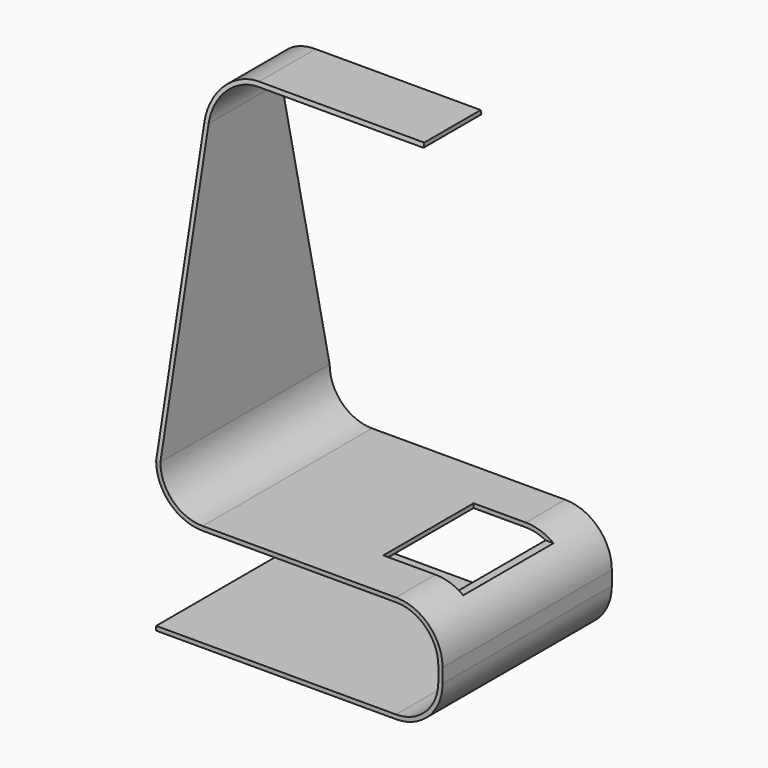
from build123d import *

# Parameters (mm, degrees)
F1_DEPTH = 75
F3_DEPTH = 200
F4_W     = 37
F4_H     = 40
F4_W_2   = 33
F5_DEPTH = 6.5


# Not quite as in the source:
# - a feature names something its author has since deleted; it is built from what else it names


with BuildPart() as f1:
    # F0 (on Front) → F1 (new body, symmetric)
    with BuildSketch(Plane.XZ):
        with BuildLine():
            Line((-67, 35), (70, 35))
            ThreePointArc((70, 35), (91.2132034356, 26.2132034356), (100, 5))
            Line((100, 5), (100, -5))
            ThreePointArc((100, -5), (91.2132034356, -26.2132034356), (70, -35))
            Line((70, -35), (-100, -35))
            Line((-100, -35), (-100, -38))
            Line((-100, -38), (70, -38))
            ThreePointArc((70, -38), (93.3345237792, -28.3345237792), (103, -5))
            Line((103, -5), (103, 5))
            ThreePointArc((103, 5), (93.3345237792, 28.3345237792), (70, 38))
            Line((70, 38), (-67, 38))
            ThreePointArc((-67, 38), (-88.2132034356, 46.7867965644), (-97, 68))
            Line((-97, 68), (-97, 262))
            ThreePointArc((-97, 262), (-88.2132034356, 283.2132034356), (-67, 292))
            Line((-67, 292), (50, 292))
            Line((50, 292), (50, 295))
            Line((50, 295), (-67, 295))
            ThreePointArc((-67, 295), (-90.3345237792, 285.3345237792), (-100, 262))
            Line((-100, 262), (-100, 68))
            ThreePointArc((-100, 68), (-90.3345237792, 44.6654762208), (-67, 35))
        make_face()
    extrude(amount=F1_DEPTH, both=True)

    # F2 (on face) → F3 (cut)
    with BuildSketch(Plane(origin=(-100, 0, 0), x_dir=(0, -1, 0), z_dir=(-1, 0, 0))):
        Polygon((-32.268722467, 262), (-75, 262), (-75, 68), align=None)
        Polygon((-75, 295), (-75, 262), (-32.268722467, 262), (-25, 295), align=None)
        Polygon((25, 295), (32.268722467, 262), (75, 262), (75, 295), align=None)
        Polygon((32.268722467, 262), (75, 68), (75, 262), align=None)
    extrude(amount=-F3_DEPTH, mode=Mode.SUBTRACT)

    # F4 (on face) → F5 (cut, symmetric)
    with BuildSketch(Plane.XY.offset(38)):
        with Locations((51.5, -20)):
            Rectangle(F4_W, F4_H)
        with Locations((86.5, -20)):
            Rectangle(F4_W_2, F4_H)
        with Locations((86.5, 20)):
            Rectangle(F4_W_2, F4_H)
        with Locations((51.5, 20)):
            Rectangle(F4_W, F4_H)
    extrude(amount=F5_DEPTH, both=True, mode=Mode.SUBTRACT)


solid = f1.part
